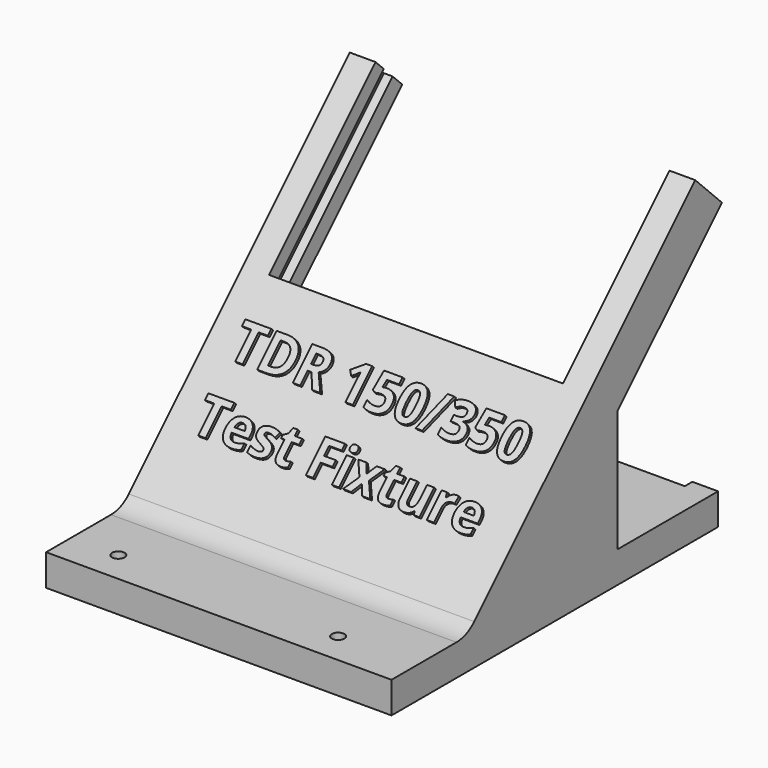
from build123d import *

# Parameters (mm, degrees)
F1_DEPTH      = 139.7
F2_W          = 118.872
F2_H          = 76.2
F3_DEPTH      = 100.1547421852
F4_R          = 2.54
F5_DEPTH      = 12.701
F6_W          = 122.428
F6_H          = 6.35
F6_W_2        = 3.556
F7_DEPTH      = 76.2
F8_W          = 132.08
F8_H          = 157.48
F8_R          = 6.35
F9_DEPTH      = 7.62
F10_T         = 5.08
F10_T3_DEPTH  = 16.002
F10_T5_DEPTH  = 13.716
F10_T7_DEPTH  = 16.51
F10_T9_DEPTH  = 18.6695337987
F10_T11_DEPTH = 13.716
F10_T13_DEPTH = 16.51
F10_T15_DEPTH = 149.86
F10_T17_DEPTH = 20.574
F10_T19_DEPTH = 20.574
F10_T21_DEPTH = 86.36
F10_T23_DEPTH = 17.78
F10_T25_DEPTH = 15.5711781649
F11_TEXT_SIZE = 19.4667690182
F12_DEPTH     = 1.27


# Not quite as in the source:
# - a shell that OpenCascade refuses in one call is made with other operations: the cavity is built on its own and cut out
# - Text() gives the source's letters only with a copy of the font that has no kerning and outlines rounded to 1/6400 em; it was checked with that copy


with BuildPart() as f1:
    # F0 (on Right) → F1 (new body)
    with BuildSketch(Plane.YZ):
        with BuildLine():
            Line((0, 12.7), (0, 0))
            Line((0, 0), (165.1, 0))
            Line((165.1, 0), (165.1, 12.7))
            Line((165.1, 12.7), (114.3250545427, 12.7))
            Line((114.3250545427, 12.7), (114.3250545427, 61.9842861795))
            Line((114.3250545427, 61.9842861795), (167.0387805207, 114.6980121575))
            Line((167.0387805207, 114.6980121575), (153.5683963391, 128.1683963391))
            Line((153.5683963391, 128.1683963391), (145.8630734528, 120.4630734528))
            Line((145.8630734528, 120.4630734528), (41.8197438789, 16.4197438789))
            ThreePointArc((41.8197438789, 16.4197438789), (37.6995673489, 13.6667299371), (32.8394877579, 12.7))
            Line((32.8394877579, 12.7), (0, 12.7))
        make_face()
    extrude(amount=F1_DEPTH)

    # F2 (on face) → F3 (cut, through all)
    with BuildSketch(Plane(origin=(0, 12.7, -12.7), x_dir=(1, 0, 0), z_dir=(0, -0.7071067812, 0.7071067812))):
        with Locations((69.85, 161.1179966125)):
            Rectangle(F2_W, F2_H)
    extrude(amount=-F3_DEPTH, mode=Mode.SUBTRACT)

    # F4 (on face) → F5 (cut, through all)
    with BuildSketch(Plane.XY.offset(12.7)):
        with Locations((19.05, 12.7)):
            Circle(F4_R)
        with Locations((107.95, 12.7)):
            Circle(F4_R)
    extrude(amount=-F5_DEPTH, mode=Mode.SUBTRACT)

    # F6 (on face) → F7 (cut)
    with BuildSketch(Plane(origin=(0, 140.8683963391, 140.8683963391), x_dir=(1, 0, 0), z_dir=(0, 0.7071067812, 0.7071067812))):
        with Locations((68.072, 26.9775122421)):
            Rectangle(F6_W, F6_H)
        with Locations((131.064, 26.9775122421)):
            Rectangle(F6_W_2, F6_H)
    extrude(amount=-F7_DEPTH, mode=Mode.SUBTRACT)

    # F8 (on face) → F9 (cut)
    with BuildSketch(Plane(origin=(0, 0, 0), x_dir=(1, 0, 0), z_dir=(0, 0, -1))):
        with Locations((69.85, -82.55)):
            Rectangle(F8_W, F8_H)
        with Locations((19.05, -12.7)):
            Circle(F8_R, mode=Mode.SUBTRACT)
        with Locations((107.95, -12.7)):
            Circle(F8_R, mode=Mode.SUBTRACT)
    extrude(amount=-F9_DEPTH, mode=Mode.SUBTRACT)

    # F10: shell of thickness 5.08, made by hand


with BuildPart() as f10_core1:
    # F10_t2: copy of F1
    add(f1.part)

    # the walls: a layer under each face that stays
    f10_faces = [f10_core1.faces().sort_by_distance(p)[0] for p in [
        (69.85, 97.694070109, 72.294070109),
        (69.85, 37.6995673489, 13.6667299371),
        (139.7, 83.5193902604, 21.3613993899),
        (134.493, 160.3035884299, 121.4332042483),
        (129.286, 128.6930868838, 99.1621690681),
        (69.85, 107.0059570777, 66.9677621477),
        (10.414, 128.6930868838, 99.1621690681),
        (5.207, 160.3035884299, 121.4332042483),
        (0, 83.5193902604, 21.3613993899),
        (69.85, 16.4197438789, 12.7),
        (69.85, 0, 6.35),
        (137.975308642, 139.303125, 0),
        (69.85, 165.1, 6.35),
        (69.85, 139.7125272714, 12.7),
        (69.85, 114.3250545427, 37.3421430898),
        (134.493, 140.6819175317, 88.3411491685),
        (129.286, 138.257248379, 89.5980075728),
        (131.064, 135.2486738521, 92.6065820997),
        (132.842, 133.0036098219, 94.85164613),
        (131.064, 130.7585457916, 97.0967101602),
        (8.636, 130.7585457916, 97.0967101602),
        (6.858, 133.0036098219, 94.85164613),
        (8.636, 135.2486738521, 92.6065820997),
        (10.414, 138.257248379, 89.5980075728),
        (5.207, 140.6819175317, 88.3411491685),
        (105.41, 12.7, 6.35),
        (16.51, 12.7, 6.35),
        (3.81, 82.55, 3.81),
        (69.85, 3.81, 3.81),
        (135.89, 82.55, 3.81),
        (69.85, 161.29, 3.81),
        (10.414, 164.1434298064, 11.7434298064),
        (69.85, 163.1868596127, 10.7868596127),
        (129.286, 164.1434298064, 11.7434298064),
        (112.1833333333, 8.4666666667, 0),
        (23.2833333333, 8.4666666667, 0),
        (101.6, 12.7, 3.81),
        (12.7, 12.7, 3.81),
    ]]
    thicken(f10_faces, amount=-F10_T, mode=Mode.SUBTRACT)

    # F10_s4 → F10_t3 (cut)
    with BuildSketch(Plane(origin=(0, 9.1078975516, -9.1078975516), x_dir=(1, 0, 0), z_dir=(0, 0.7071067812, -0.7071067812))):
        Polygon((129.2352, -123.0687966125), (134.366, -123.0179966125), (134.366, -117.9379966125), (129.286, -117.9379966125), align=None)
        Polygon((10.4648, -123.0687966125), (10.414, -117.9379966125), (5.334, -117.9379966125), (5.334, -123.0179966125), align=None)
    extrude(amount=F10_T3_DEPTH, mode=Mode.SUBTRACT)

    # F10_s6 → F10_t5 (cut)
    with BuildSketch(Plane.YZ.offset(1.778)):
        Polygon((103.8896194774, 70.155941797), (100.22567498, 66.5638393486), (96.6335725315, 70.155941797), (100.22567498, 73.7480442454), align=None)
        Polygon((108.3079054889, 65.7376557854), (104.7158030405, 62.0737112881), (108.3079054889, 58.4816088396), (111.9000079374, 62.0737112881), align=None)
    extrude(amount=F10_T5_DEPTH, mode=Mode.SUBTRACT)

    # F10_s8 → F10_t7 (cut)
    with BuildSketch(Plane(origin=(0, 24.9131483247, -24.9131483247), x_dir=(1, 0, 0), z_dir=(0, -0.7071067812, 0.7071067812))):
        Polygon((6.9088, 123.0687966125), (6.858, 117.9379966125), (1.778, 117.9379966125), (1.778, 123.0179966125), align=None)
    extrude(amount=F10_T7_DEPTH, mode=Mode.SUBTRACT)

    # F10_s10 → F10_t9 (cut)
    with BuildSketch(Plane(origin=(0, 17.7289434278, -17.7289434278), x_dir=(1, 0, 0), z_dir=(0, 0.7071067812, -0.7071067812))):
        Polygon((10.4648, -123.0687966125), (10.414, -117.9379966125), (5.334, -117.9379966125), (5.334, -123.0179966125), align=None)
        Polygon((129.2352, -123.0687966125), (129.286, -117.9379966125), (134.366, -117.9379966125), (134.366, -123.0179966125), align=None)
    extrude(amount=F10_T9_DEPTH, mode=Mode.SUBTRACT)

    # F10_s12 → F10_t11 (cut)
    with BuildSketch(Plane.YZ.offset(124.206)):
        Polygon((108.3079054889, 65.7376557854), (104.7158030405, 62.0737112881), (108.3079054889, 58.4816088396), (111.9000079374, 62.0737112881), align=None)
        Polygon((103.8896194774, 70.155941797), (100.22567498, 66.5638393486), (96.6335725315, 70.155941797), (100.22567498, 73.7480442454), align=None)
    extrude(amount=F10_T11_DEPTH, mode=Mode.SUBTRACT)

    # F10_s14 → F10_t13 (cut)
    with BuildSketch(Plane(origin=(0, 13.2388153673, -13.2388153673), x_dir=(1, 0, 0), z_dir=(0, 0.7071067812, -0.7071067812))):
        Polygon((132.7912, -123.0687966125), (132.842, -117.9379966125), (137.922, -117.9379966125), (137.922, -123.0179966125), align=None)
    extrude(amount=F10_T13_DEPTH, mode=Mode.SUBTRACT)

    # F10_s16 → F10_t15 (cut)
    with BuildSketch(Plane.YZ.offset(-5.08)):
        Polygon((114.3758545427, 12.7508), (114.3250545427, 7.62), (109.2450545427, 7.62), (109.2450545427, 12.7), align=None)
    extrude(amount=F10_T15_DEPTH, mode=Mode.SUBTRACT)

    # F10_s18 → F10_t17 (cut)
    with BuildSketch(Plane.YZ.offset(-5.08)):
        Polygon((114.4117755672, 61.9483651551), (109.2450545427, 61.9842861795), (109.2450545427, 64.0884910764), (110.7329520943, 65.576388628), align=None)
    extrude(amount=F10_T17_DEPTH, mode=Mode.SUBTRACT)

    # F10_s20 → F10_t19 (cut)
    with BuildSketch(Plane.YZ.offset(124.206)):
        Polygon((114.4117755672, 61.9483651551), (109.2450545427, 61.9842861795), (109.2450545427, 64.0884910764), (110.7329520943, 65.576388628), align=None)
    extrude(amount=F10_T19_DEPTH, mode=Mode.SUBTRACT)

    # F10_s22 → F10_t21 (cut)
    with BuildSketch(Plane(origin=(0, 144.4604987875, 144.4604987875), x_dir=(1, 0, 0), z_dir=(0, -0.7071067812, -0.7071067812))):
        Polygon((132.7912, -30.1017122421), (132.842, -35.2325122421), (137.922, -35.2325122421), (137.922, -30.1525122421), align=None)
        Polygon((132.7912, -23.8533122421), (137.922, -23.8025122421), (137.922, -18.7225122421), (132.842, -18.7225122421), align=None)
        Polygon((6.9088, -23.8533122421), (6.858, -18.7225122421), (1.778, -18.7225122421), (1.778, -23.8025122421), align=None)
        Polygon((6.9088, -30.1017122421), (1.778, -30.1525122421), (1.778, -35.2325122421), (6.858, -35.2325122421), align=None)
    extrude(amount=F10_T21_DEPTH, mode=Mode.SUBTRACT)

    # F10_s24 → F10_t23 (cut)
    with BuildSketch(Plane.XY.offset(-5.08)):
        Polygon((3.8608, 3.8608), (-1.27, 3.81), (-1.27, -1.27), (3.81, -1.27), align=None)
        Polygon((3.8608, 161.2392), (-1.27, 161.29), (-1.27, 166.37), (3.81, 166.37), align=None)
        Polygon((135.8392, 3.8608), (135.89, -1.27), (140.97, -1.27), (140.97, 3.81), align=None)
        Polygon((135.8392, 161.2392), (140.97, 161.29), (140.97, 166.37), (135.89, 166.37), align=None)
    extrude(amount=F10_T23_DEPTH, mode=Mode.SUBTRACT)

    # F10_s26 → F10_t25 (cut)
    with BuildSketch(Plane(origin=(0, 70.6947571643, -70.6947571643), x_dir=(1, 0, 0), z_dir=(0, 0.7071067812, -0.7071067812))):
        Polygon((10.4648, -123.0687966125), (5.334, -123.0179966125), (5.334, -117.9379966125), (10.414, -117.9379966125), align=None)
        Polygon((129.2352, -123.0687966125), (129.286, -117.9379966125), (134.366, -117.9379966125), (134.366, -123.0179966125), align=None)
    extrude(amount=F10_T25_DEPTH, mode=Mode.SUBTRACT)


with BuildPart() as f1_1:
    add(f1.part)

    # what is left inside the walls is the cavity
    f10_cavity = [f10_core1.part.solids().sort_by_distance(p)[0] for p in [
        (91.44, 72.585274, 39.929227),
    ]]
    add(f10_cavity, mode=Mode.SUBTRACT)

    # F11 (on face) → F12 (join)
    with BuildSketch(Plane(origin=(0, 12.7, -12.7), x_dir=(1, 0, 0), z_dir=(0, -0.7071067812, 0.7071067812))):
        with Locations((10.414, 92.822486728)):
            Text('TDR 150/350', F11_TEXT_SIZE, font='Open Sans', font_style=FontStyle.BOLD, text_align=(TextAlign.LEFT, TextAlign.BOTTOM))
        with Locations((10.414, 66.3476808633)):
            Text('Test Fixture', F11_TEXT_SIZE, font='Open Sans', font_style=FontStyle.BOLD, text_align=(TextAlign.LEFT, TextAlign.BOTTOM))
    extrude(amount=F12_DEPTH)


solid = f1_1.part
